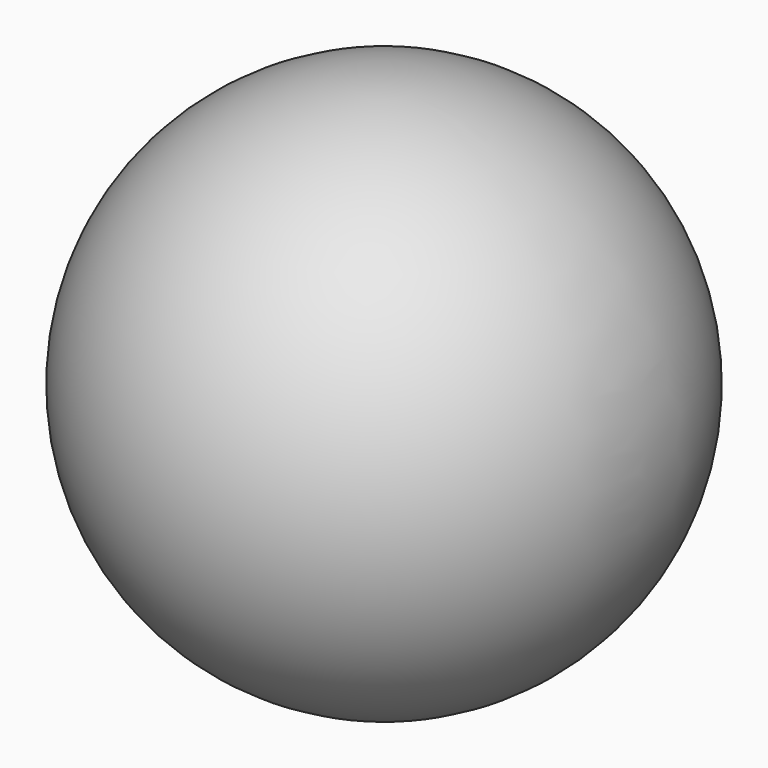
from build123d import *

# Parameters (mm, degrees)
F2_R     = 3.175
F3_DEPTH = 101.6


# Not quite as in the source:
# - a fillet or chamfer that OpenCascade refuses, or shapes differently, is made with other operations: its cross-section is extruded or revolved along the edge and cut away or added


with BuildPart() as f1:
    # F0 (on Front) → F1 (revolve)
    with BuildSketch(Plane.XZ):
        with BuildLine():
            ThreePointArc((0, -50.8), (50.8, 0), (0, 50.8))
            Line((0, 50.8), (0, 44.45))
            ThreePointArc((0, 44.45), (44.45, 0), (0, -44.45))
            Line((0, -44.45), (0, -50.8))
        make_face()
    revolve(axis=Axis((0, 0, 0), (0, 0, -1)))

    # F2 (on Front) → F3 (cut)
    with BuildSketch(Plane.XZ):
        Circle(F2_R)
    extrude(amount=-F3_DEPTH, mode=Mode.SUBTRACT)

    # F4: chamfer of 6.35 on 1 edges, made by hand

    # F4_s1 → F4_t2 (revolve, cut)
    with BuildSketch(Plane.XY.offset(-1.2e-09)):
        with BuildLine():
            Line((3.0138514094, 50.4834593112), (8.8272948956, 43.4006886388))
            Line((8.8272948956, 43.4006886388), (8.8025344773, 43.2761257162))
            ThreePointArc((8.8025344773, 43.2761257162), (6.0073622852, 43.914006044), (3.1659285713, 44.2097865329))
            Line((3.1659285713, 44.2097865329), (3.048, 44.336462139))
            ThreePointArc((3.048, 44.336462139), (3.047999955, 47.4099607251), (2.8868514094, 50.4834593112))
            Line((2.8868514094, 50.4834593112), (3.0138514094, 50.4834593112))
        make_face()
    revolve(axis=Axis((-2.25e-08, 44.336462139, -1.2e-09), (0, -1, 0)), mode=Mode.SUBTRACT)


solid = f1.part
